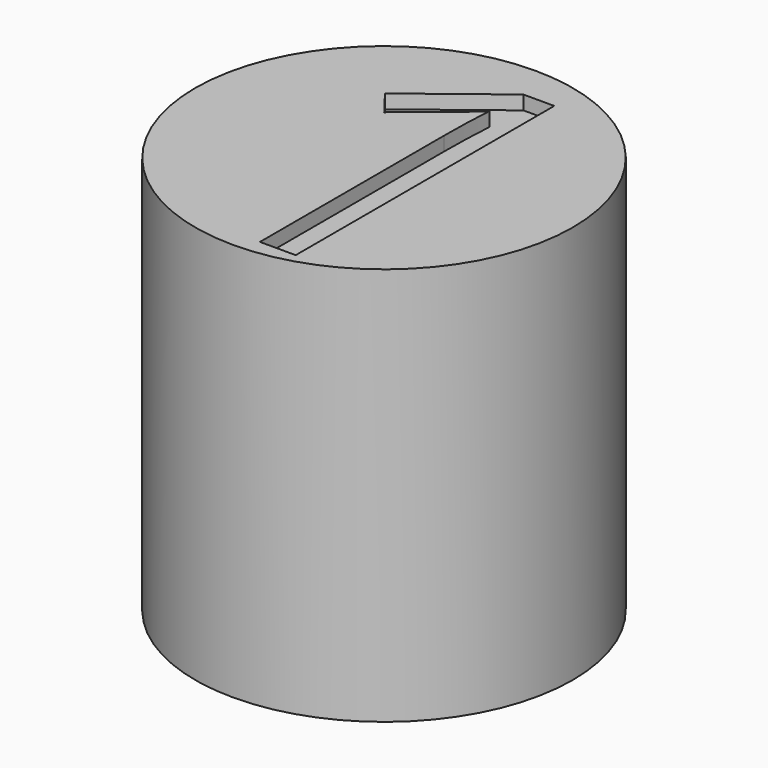
from build123d import *

# Parameters (mm, degrees)
F1_R         = 13.5
F2_DEPTH     = 28.49
F3_TEXT_SIZE = 32.3697466089
F4_DEPTH     = 1


# Not quite as in the source:
# - Text() gives the source's letters only with a copy of the font that has no kerning and outlines rounded to 1/6400 em; it was checked with that copy


with BuildPart() as f2:
    # F1 (on Top) → F2 (new body)
    with BuildSketch(Plane.XY):
        Circle(F1_R)
    extrude(amount=F2_DEPTH)

    # F3 (on face) → F4 (cut)
    with BuildSketch(Plane.XY.offset(28.49)):
        with Locations((-7.788139388, -12.2792104906)):
            Text('1', F3_TEXT_SIZE, font='Open Sans', text_align=(TextAlign.LEFT, TextAlign.BOTTOM))
    extrude(amount=-F4_DEPTH, mode=Mode.SUBTRACT)


solid = f2.part
